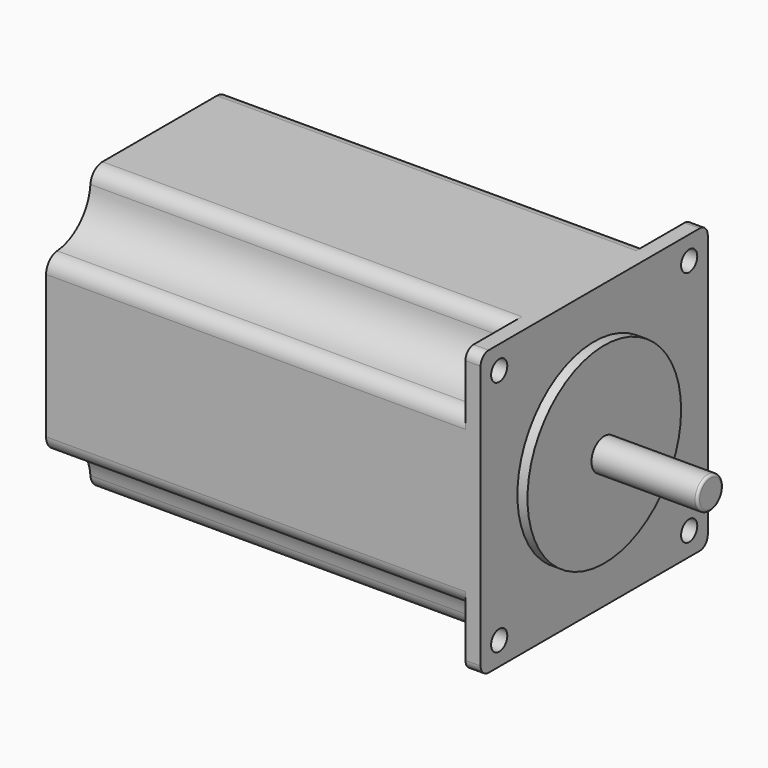
from build123d import *

# Parameters (mm, degrees)
F0_R     = 2
F1_DEPTH = 86
F2_R     = 19
F3_DEPTH = 2
F4_R     = 3.175
F5_DEPTH = 21
F6_R     = 0.5
F8_R     = 9
F9_DEPTH = 83
F10_R    = 3


# Not quite as in the source:
# - a feature names something its author has since deleted; it is built from what else it names


with BuildPart() as f1:
    # F0 (on Right) → F1 (new body)
    with BuildSketch(Plane.YZ):
        with BuildLine():
            Line((26.1, 28.1), (-26.1, 28.1))
            ThreePointArc((-26.1, 28.1), (-27.5142135624, 27.5142135624), (-28.1, 26.1))
            Line((-28.1, 26.1), (-28.1, -26.1))
            ThreePointArc((-28.1, -26.1), (-27.5142135624, -27.5142135624), (-26.1, -28.1))
            Line((-26.1, -28.1), (26.1, -28.1))
            ThreePointArc((26.1, -28.1), (27.5142135624, -27.5142135624), (28.1, -26.1))
            Line((28.1, -26.1), (28.1, 26.1))
            ThreePointArc((28.1, 26.1), (27.5142135624, 27.5142135624), (26.1, 28.1))
        make_face()
        with Locations((-23.5, -23.5)):
            Circle(F0_R, mode=Mode.SUBTRACT)
        with Locations((23.5, -23.5)):
            Circle(F0_R, mode=Mode.SUBTRACT)
        with Locations((-23.5, 23.5)):
            Circle(F0_R, mode=Mode.SUBTRACT)
        with Locations((23.5, 23.5)):
            Circle(F0_R, mode=Mode.SUBTRACT)
    extrude(amount=F1_DEPTH)

    # F2 (on face) → F3 (join)
    with BuildSketch(Plane.YZ.offset(86)):
        Circle(F2_R)
    extrude(amount=F3_DEPTH)

    # F4 (on face) → F5 (join)
    with BuildSketch(Plane.YZ.offset(88)):
        Circle(F4_R)
    extrude(amount=F5_DEPTH)

    # F6
    f6_edges = [f1.edges().sort_by_distance(p)[0] for p in [
        (109, -3.175, 0),
    ]]
    fillet(f6_edges, radius=F6_R)

    # F8 (on offset) → F9 (cut, through all)
    with BuildSketch(Plane.YZ.offset(83)):
        with Locations((-26.1, 26.1)):
            Circle(F8_R)
        with Locations((26.1, 26.1)):
            Circle(F8_R)
        with Locations((-26.1, -26.1)):
            Circle(F8_R)
        with Locations((26.1, -26.1)):
            Circle(F8_R)
    extrude(amount=-F9_DEPTH, mode=Mode.SUBTRACT)

    # F10
    f10_edges = [f1.edges().sort_by_distance(p)[0] for p in [
        (41.5, 17.325036, 28.1),
        (41.5, 28.1, 17.325036),
        (41.5, -17.325036, 28.1),
        (41.5, -28.1, 17.325036),
        (41.5, -28.1, -17.325036),
        (41.5, -17.325036, -28.1),
        (41.5, 17.325036, -28.1),
        (41.5, 28.1, -17.325036),
    ]]
    fillet(f10_edges, radius=F10_R)


solid = f1.part
